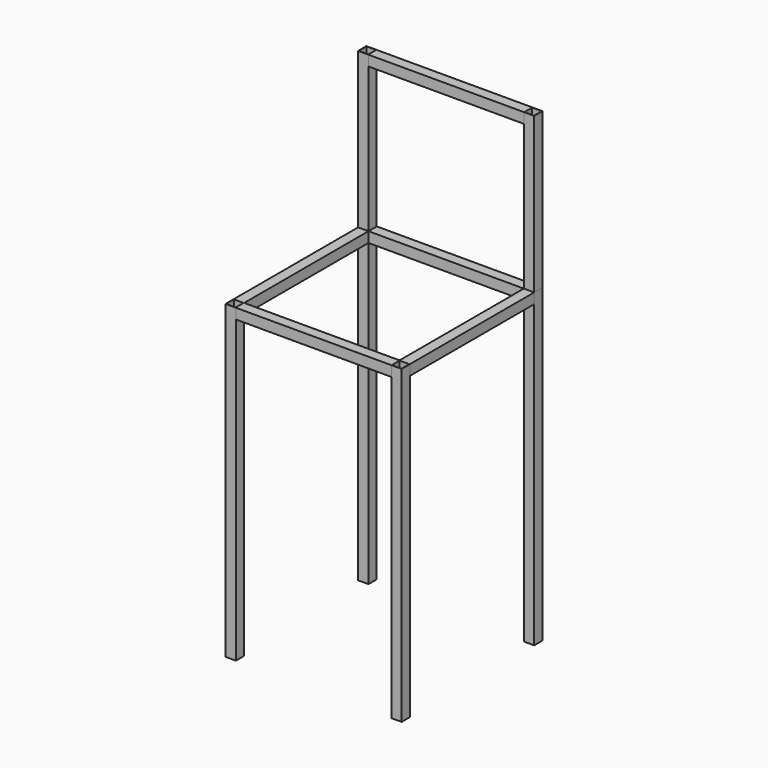
from build123d import *

# Parameters (mm, degrees)
F0_W      = 25.4
F0_H      = 25.4
F0_W_2    = 23.8125
F0_H_2    = 23.8125
F1_DEPTH  = 1143
F0_W_3    = 23.8252
F2_W      = 25.4
F2_H      = 25.4
F3_DEPTH  = 381
F7_DEPTH  = 762
F8_W      = 25.4
F8_H      = 25.4
F9_DEPTH  = 381
F10_W     = 25.4
F10_H     = 38.2154002551
F11_DEPTH = 381
F10_H_2   = 25.4
F14_DEPTH = 381


# Not quite as in the source:
# - the program builds the solid bodies; features that only make, move or delete a surface that nothing else refers to are left out


with BuildPart() as f1:
    # F0 (on Top) → F1 (new body)
    with BuildSketch(Plane.XY):
        with Locations((-203.2, 0)):
            Rectangle(F0_W, F0_H)
        with Locations((-203.2, 0)):
            Rectangle(F0_W_2, F0_H_2, mode=Mode.SUBTRACT)
    extrude(amount=F1_DEPTH)


with BuildPart() as f1b:
    # F0 (on Top) → F1, piece 2 (new body)
    with BuildSketch(Plane.XY):
        with Locations((203.2, 0)):
            Rectangle(F0_W, F0_H)
        with Locations((203.2, 0)):
            Rectangle(F0_W_2, F0_H_2, mode=Mode.SUBTRACT)
    extrude(amount=F1_DEPTH)


with BuildPart() as f1c:
    # F0 (on Top) → F1, piece 3 (new body)
    with BuildSketch(Plane.XY):
        with Locations((-203.2, -406.4)):
            Rectangle(F0_W, F0_H)
        with Locations((-203.2, -406.4)):
            Rectangle(F0_W_3, F0_H_2, mode=Mode.SUBTRACT)
    extrude(amount=F1_DEPTH)


with BuildPart() as f1d:
    # F0 (on Top) → F1, piece 4 (new body)
    with BuildSketch(Plane.XY):
        with Locations((203.2, -406.4)):
            Rectangle(F0_W, F0_H)
        with Locations((203.2, -406.4)):
            Rectangle(F0_W_3, F0_H_2, mode=Mode.SUBTRACT)
    extrude(amount=F1_DEPTH)


with BuildPart() as f3:
    # F2 (on face) → F3 (new body)
    with BuildSketch(Plane.XZ.offset(12.7)):
        with Locations((-203.2, 749.3)):
            Rectangle(F2_W, F2_H)
    extrude(amount=F3_DEPTH)


with BuildPart() as f4_1:
    # F4: instance of F3
    add(f3.part.mirror(Plane.YZ))


with BuildPart() as f7:
    # F0 (on Top) → F7 (new body)
    with BuildSketch(Plane.XY):
        with Locations((-203.2, 0)):
            Rectangle(F0_W, F0_H)
        with Locations((-203.2, 0)):
            Rectangle(F0_W_2, F0_H_2, mode=Mode.SUBTRACT)
    extrude(amount=F7_DEPTH)


with BuildPart() as f7b:
    # F0 (on Top) → F7, piece 2 (new body)
    with BuildSketch(Plane.XY):
        with Locations((203.2, 0)):
            Rectangle(F0_W, F0_H)
        with Locations((203.2, 0)):
            Rectangle(F0_W_2, F0_H_2, mode=Mode.SUBTRACT)
    extrude(amount=F7_DEPTH)


with BuildPart() as f7c:
    # F0 (on Top) → F7, piece 3 (new body)
    with BuildSketch(Plane.XY):
        with Locations((-203.2, -406.4)):
            Rectangle(F0_W, F0_H)
        with Locations((-203.2, -406.4)):
            Rectangle(F0_W_3, F0_H_2, mode=Mode.SUBTRACT)
    extrude(amount=F7_DEPTH)


with BuildPart() as f7d:
    # F0 (on Top) → F7, piece 4 (new body)
    with BuildSketch(Plane.XY):
        with Locations((203.2, -406.4)):
            Rectangle(F0_W, F0_H)
        with Locations((203.2, -406.4)):
            Rectangle(F0_W_3, F0_H_2, mode=Mode.SUBTRACT)
    extrude(amount=F7_DEPTH)


with BuildPart() as f9:
    # F8 (on face) → F9 (new body)
    with BuildSketch(Plane.YZ.offset(-190.5)):
        with Locations((-406.4, 749.3)):
            Rectangle(F8_W, F8_H)
    extrude(amount=F9_DEPTH)


with BuildPart() as f11:
    # F10 (on face) → F11 (new body)
    with BuildSketch(Plane.YZ.offset(-190.5)):
        with Locations((0, 1047.0973100239)):
            Rectangle(F10_W, F10_H)
    extrude(amount=F11_DEPTH)


with BuildPart() as f11b:
    # F10 (on face) → F11, piece 2 (new body)
    with BuildSketch(Plane.YZ.offset(-190.5)):
        with Locations((0, 749.3)):
            Rectangle(F10_W, F10_H_2)
    extrude(amount=F11_DEPTH)


with BuildPart() as f14:
    # F13 (on face) → F14 (new body)
    with BuildSketch(Plane.YZ.offset(-190.5)):
        Polygon((12.7, 1117.6), (12.7, 1143), (-12.7, 1143), (-12.7, 1117.6), (-11.1125, 1117.6), align=None)
    extrude(amount=F14_DEPTH)


solid = Compound([f1.part, f1b.part, f3.part, f4_1.part, f7.part, f7b.part, f7c.part, f7d.part, f9.part, f11b.part, f14.part])
